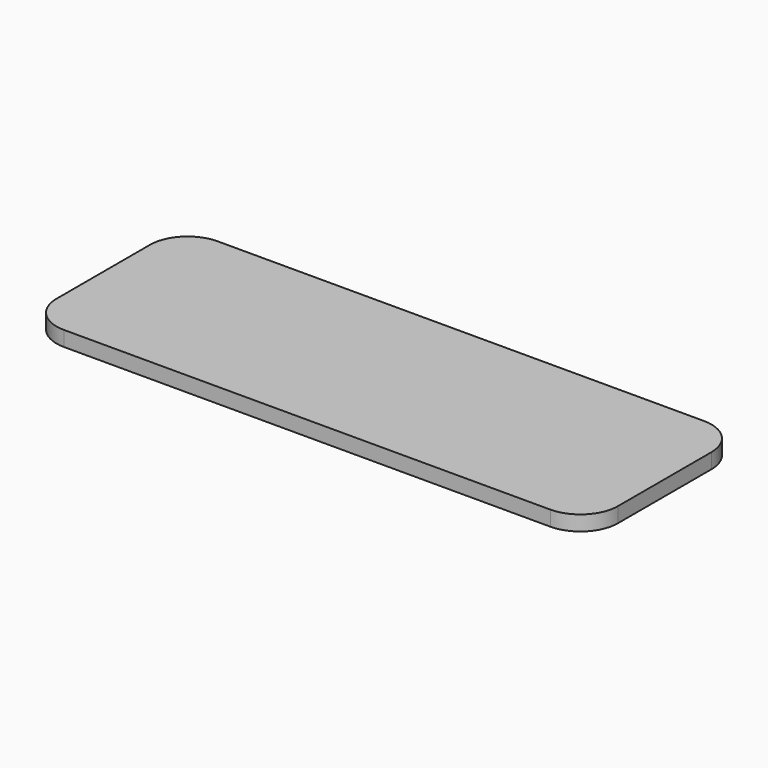
from build123d import *

# Parameters (mm, degrees)
F1_DEPTH = 2


# Not quite as in the source:
# - the program builds the solid bodies; features that only make, move or delete a surface that nothing else refers to are left out


with BuildPart() as f1:
    # F0 (on Top) → F1 (new body)
    with BuildSketch(Plane.XY):
        with BuildLine():
            Line((33.1883379823, 11.9417690091), (-31.4066620177, 11.9417690091))
            ThreePointArc((-31.4066620177, 11.9417690091), (-34.9421959236, 10.477302915), (-36.4066620177, 6.9417690091))
            Line((-36.4066620177, 6.9417690091), (-36.4066620177, -8.5672309909))
            ThreePointArc((-36.4066620177, -8.5672309909), (-34.9421959236, -12.1027648969), (-31.4066620177, -13.5672309909))
            Line((-31.4066620177, -13.5672309909), (33.1883379823, -13.5672309909))
            ThreePointArc((33.1883379823, -13.5672309909), (36.7238718882, -12.1027648969), (38.1883379823, -8.5672309909))
            Line((38.1883379823, -8.5672309909), (38.1883379823, 6.9417690091))
            ThreePointArc((38.1883379823, 6.9417690091), (36.7238718882, 10.477302915), (33.1883379823, 11.9417690091))
        make_face()
    extrude(amount=F1_DEPTH)


solid = f1.part
